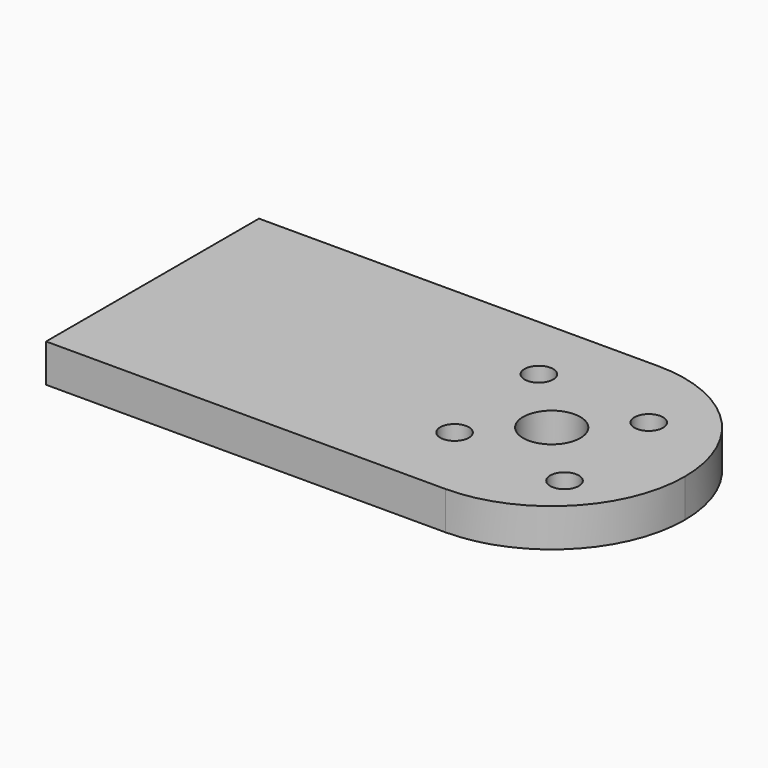
from build123d import *

# Parameters (mm, degrees)
F0_W     = 55.8
F0_H     = 27.9
F0_R     = 1.5
F0_R_2   = 3
F1_DEPTH = 4
F2_R     = 13.94999


# Not quite as in the source:
# - a fillet or chamfer is up to 0.001 mm smaller than in the source, because OpenCascade refuses the exact size


with BuildPart() as f1:
    # F0 (on Top) → F1 (new body)
    with BuildSketch(Plane.XY):
        with Locations((-27.9, 13.95)):
            Rectangle(F0_W, F0_H)
        with Locations((-19.6068542495, 8.2931457505)):
            Circle(F0_R, mode=Mode.SUBTRACT)
        with Locations((-7.2324855787, 7.2324855787)):
            Circle(F0_R, mode=Mode.SUBTRACT)
        with Locations((-20.6675144213, 20.6675144213)):
            Circle(F0_R, mode=Mode.SUBTRACT)
        with Locations((-13.95, 13.95)):
            Circle(F0_R_2, mode=Mode.SUBTRACT)
        with Locations((-8.2931457505, 19.6068542495)):
            Circle(F0_R, mode=Mode.SUBTRACT)
    extrude(amount=F1_DEPTH)

    # F2 (radius 13.95 in the source; OpenCascade refuses exactly that, so slightly less here)
    f2_edges = [f1.edges().sort_by_distance(p)[0] for p in [
        (0, 27.9, 2),
        (0, 0, 2),
    ]]
    fillet(f2_edges, radius=F2_R)


solid = f1.part
